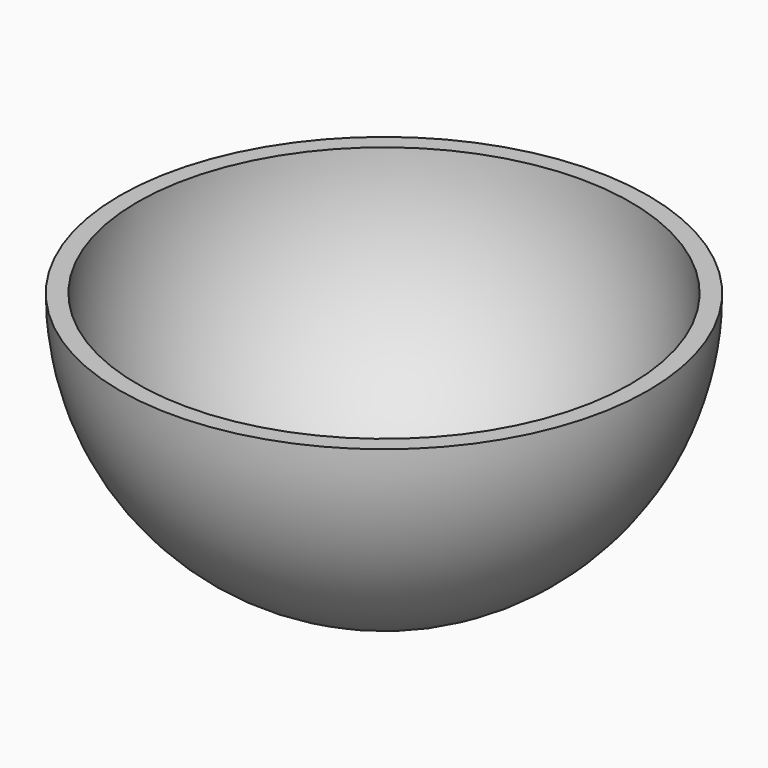
from build123d import *

# Parameters (mm, degrees)
F1_ANGLE = 180


with BuildPart() as f1:
    # F0 (on Top) → F1 (revolve)
    with BuildSketch(Plane.XY):
        with BuildLine():
            ThreePointArc((-95.25, 0), (0, -95.25), (95.25, 0))
            Line((95.25, 0), (88.9, 0))
            ThreePointArc((88.9, 0), (0, -88.9), (-88.9, 0))
            Line((-88.9, 0), (-95.25, 0))
        make_face()
    revolve(axis=Axis((0, 0, 0), (1, 0, 0)), revolution_arc=F1_ANGLE)


solid = f1.part
